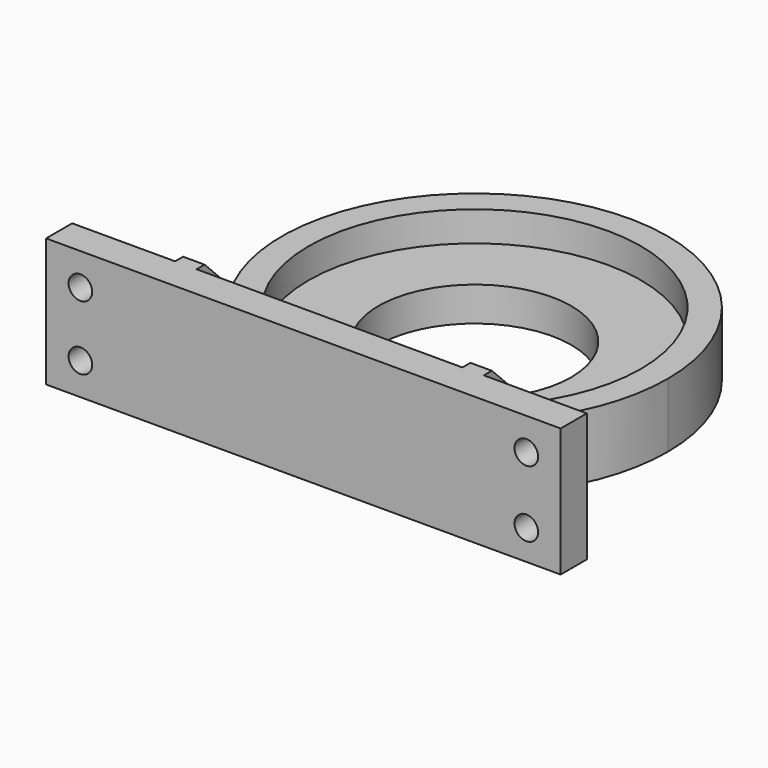
from build123d import *

# Parameters (mm, degrees)
F0_W      = 24
F0_H      = 7.6146386564
F1_DEPTH  = 15
F2_R      = 38.75
F4_DEPTH  = 7
F5_DEPTH  = 15
F7_DEPTH  = 15
F8_SIZE   = 14.99999
F9_R      = 2.75
F10_DEPTH = 25
F11_R     = 22.5
F12_DEPTH = 25


# Not quite as in the source:
# - a fillet or chamfer is up to 0.001 mm smaller than in the source, because OpenCascade refuses the exact size


with BuildPart() as f1:
    # F0 (on Top) → F1 (new body)
    with BuildSketch(Plane.XY):
        with BuildLine():
            ThreePointArc((36, -27), (42.6907484123, -14.2302494708), (45, 0))
            ThreePointArc((45, 0), (-14.2302494708, 42.6907484123), (-36, -27))
            Line((-36, -27), (36, -27))
        make_face()
        with BuildLine():
            ThreePointArc((-15.1652218257, -42.3676297069), (-26.7116265289, -36.2144861648), (-36, -27))
            Line((-36, -27), (-36, -42.3676297069))
            Line((-36, -42.3676297069), (-15.1652218257, -42.3676297069))
        make_face()
        with BuildLine():
            Line((36, -27), (-36, -27))
            ThreePointArc((-36, -27), (-26.7116265289, -36.2144861648), (-15.1652218257, -42.3676297069))
            Line((-15.1652218257, -42.3676297069), (15.1652218257, -42.3676297069))
            ThreePointArc((15.1652218257, -42.3676297069), (26.7116265289, -36.2144861648), (36, -27))
        make_face()
        with BuildLine():
            Line((15.1652218257, -42.3676297069), (-15.1652218257, -42.3676297069))
            ThreePointArc((-15.1652218257, -42.3676297069), (0, -45), (15.1652218257, -42.3676297069))
        make_face()
        with Locations((-48, -46.174949035)):
            Rectangle(F0_W, F0_H)
        with BuildLine():
            ThreePointArc((15.1652218257, -42.3676297069), (0, -45), (-15.1652218257, -42.3676297069))
            Line((-15.1652218257, -42.3676297069), (-36, -42.3676297069))
            Line((-36, -42.3676297069), (-36, -49.9822683632))
            Line((-36, -49.9822683632), (36, -49.9822683632))
            Line((36, -49.9822683632), (36, -42.3676297069))
            Line((36, -42.3676297069), (15.1652218257, -42.3676297069))
        make_face()
        with Locations((48, -46.174949035)):
            Rectangle(F0_W, F0_H)
        with BuildLine():
            Line((36, -42.3676297069), (36, -27))
            ThreePointArc((36, -27), (26.7116265289, -36.2144861648), (15.1652218257, -42.3676297069))
            Line((15.1652218257, -42.3676297069), (36, -42.3676297069))
        make_face()
    extrude(amount=F1_DEPTH)

    # F2 (on face) → F4 (cut)
    with BuildSketch(Plane.XY.offset(15)):
        Circle(F2_R)
    extrude(amount=-F4_DEPTH, mode=Mode.SUBTRACT)

    # F3 (on face) → F5 (join)
    with BuildSketch(Plane.XY.offset(15)):
        Polygon((-36, -42.3676297069), (-60, -42.3676297069), (-60, -49.9822683632), (60, -49.9822683632), (60, -42.3676297069), (36, -42.3676297069), align=None)
    extrude(amount=F5_DEPTH)

    # F6 (on face) → F7 (join)
    with BuildSketch(Plane.XY.offset(15)):
        Polygon((-31, -25.031657964), (-36, -25.031657964), (-36, -27), (-36, -42.3676297069), (-31, -42.3676297069), align=None)
        Polygon((36, -42.3676297069), (36, -27), (36, -25.031657964), (31, -25.031657964), (31, -42.3676297069), align=None)
    extrude(amount=F7_DEPTH)

    # F8 (size 15 in the source; OpenCascade refuses exactly that, so slightly less here)
    f8_edges = [f1.edges().sort_by_distance(p)[0] for p in [
        (-33.5, -25.031658, 30),
        (33.5, -25.031658, 30),
    ]]
    chamfer(f8_edges, length=F8_SIZE)

    # F9 (on face) → F10 (cut)
    with BuildSketch(Plane(origin=(0, -42.3676297069, 0), x_dir=(-1, 0, 0), z_dir=(0, 1, 0))):
        with Locations((52, 7.5)):
            Circle(F9_R)
        with Locations((52, 22.5)):
            Circle(F9_R)
        with Locations((-52, 7)):
            Circle(F9_R)
        with Locations((-52, 22.5)):
            Circle(F9_R)
    extrude(amount=-F10_DEPTH, mode=Mode.SUBTRACT)

    # F11 (on face) → F12 (cut)
    with BuildSketch(Plane.XY.offset(8)):
        Circle(F11_R)
    extrude(amount=-F12_DEPTH, mode=Mode.SUBTRACT)


solid = f1.part
